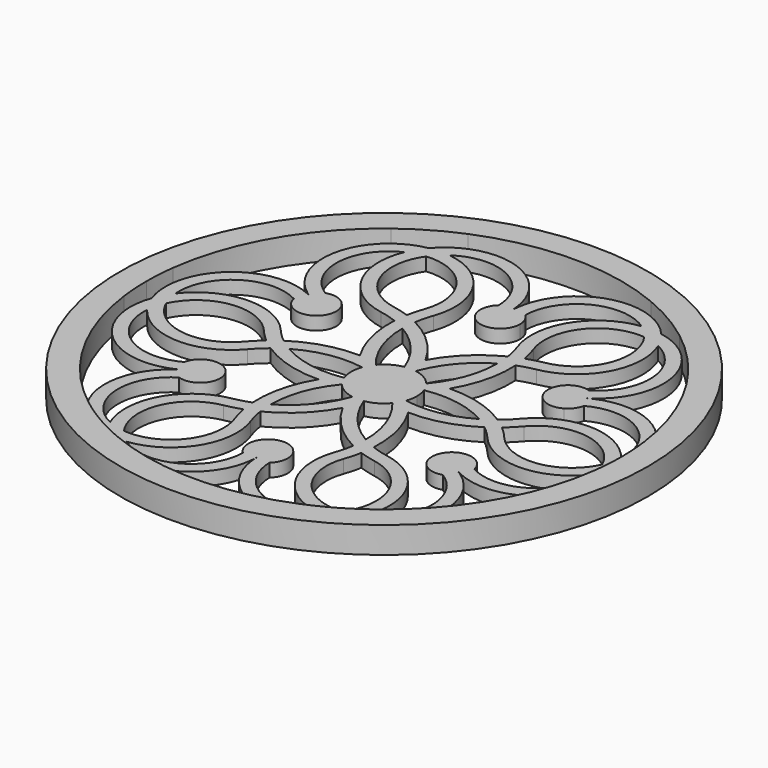
from build123d import *

# Parameters (mm, degrees)
F0_R     = 20
F2_DEPTH = 2
F3_DEPTH = 1
F4_COUNT = 6
F5_DEPTH = 1


# Not quite as in the source:
# - a feature names something its author has since deleted; it is built from what else it names


with BuildPart() as f2:
    # F0 (on Top) → F2 (new body)
    with BuildSketch(Plane.XY):
        Circle(F0_R)
        with BuildLine():
            ThreePointArc((18, 0), (-9.9846036052, -14.9769052493), (-6.9230767608, 16.615384683))
            ThreePointArc((-6.9230767608, 16.615384683), (1.3e-07, 18), (6.9230770009, 16.615384583))
            ThreePointArc((6.9230770009, 16.615384583), (14.9769053214, 9.984603497), (18, 0))
        make_face(mode=Mode.SUBTRACT)
    extrude(amount=F2_DEPTH)

    # F0 (on Top) → F3 (join)
    with BuildSketch(Plane.XY):
        with BuildLine():
            ThreePointArc((-1.0016972865, 12.1165135674), (-0.5479723364, 12.3963260072), (-0.0250418091, 12.4997909547))
            ThreePointArc((-0.0250418091, 12.4997909547), (-2.4381602314, 16.2938301084), (-6.9230767608, 16.615384683))
            ThreePointArc((-6.9230767608, 16.615384683), (-9.971545779, 11.4673344692), (-5.9016393443, 7.0819672131))
            ThreePointArc((-5.9016393443, 7.0819672131), (-2.5530323929, 5.499608355), (-0.4340277778, 2.4620357203))
            ThreePointArc((-0.4340277778, 2.4620357203), (0, 2.5), (0.4340277778, 2.4620357203))
            ThreePointArc((0.4340277778, 2.4620357203), (2.5530323929, 5.499608355), (5.9016393443, 7.0819672131))
            ThreePointArc((5.9016393443, 7.0819672131), (9.9715457651, 11.4673343399), (6.9230770009, 16.615384583))
            ThreePointArc((6.9230770009, 16.615384583), (2.4381603431, 16.293830175), (0.0250418091, 12.4997909547))
            ThreePointArc((0.0250418091, 12.4997909547), (0.5479723364, 12.3963260072), (1.0016972865, 12.1165135674))
            ThreePointArc((1.0016972865, 12.1165135674), (7.6052247894, 15.0352600872), (5.7213114754, 8.0655737705))
            ThreePointArc((5.7213114754, 8.0655737705), (2.3919359235, 6.6424784408), (0, 3.9242833741))
            ThreePointArc((0, 3.9242833741), (-2.3919359235, 6.6424784408), (-5.7213114754, 8.0655737705))
            ThreePointArc((-5.7213114754, 8.0655737705), (-7.6052247894, 15.0352600872), (-1.0016972865, 12.1165135674))
        make_face()
        with BuildLine():
            ThreePointArc((0.0250418091, 12.4997909547), (0.0062643765, 12.250208958), (0, 12))
            ThreePointArc((0, 12), (-0.0062643765, 12.250208958), (-0.0250418091, 12.4997909547))
            ThreePointArc((-0.0250418091, 12.4997909547), (-0.5479723364, 12.3963260072), (-1.0016972865, 12.1165135674))
            ThreePointArc((-1.0016972865, 12.1165135674), (-0.6113321807, 9.630228864), (1.5, 11))
            ThreePointArc((1.5, 11), (1.369771136, 11.6113321807), (1.0016972865, 12.1165135674))
            ThreePointArc((1.0016972865, 12.1165135674), (0.5479723364, 12.3963260072), (0.0250418091, 12.4997909547))
        make_face()
    extrude(amount=F3_DEPTH)

    # F4: F2 ×6 about axis
    f4_axis = Axis((0, 0, 6.8624988198), (0, 0, 1))


with BuildPart() as f2_1:
    add(f2.part)
    for i in range(1, F4_COUNT):
        add(f2.part.rotate(f4_axis, i * 360 / F4_COUNT))

    # F0 (on Top) → F5 (join)
    with BuildSketch(Plane.XY):
        with BuildLine():
            ThreePointArc((0, 0), (-0.1093371255, 1.25), (-0.4340277778, 2.4620357203))
            ThreePointArc((-0.4340277778, 2.4620357203), (-1.6070050646, -1.9150808657), (2.5, 0))
            ThreePointArc((2.5, 0), (1.9150808657, 1.6070050646), (0.4340277778, 2.4620357203))
            ThreePointArc((0.4340277778, 2.4620357203), (0.1093371255, 1.25), (0, 0))
        make_face()
        with BuildLine():
            ThreePointArc((0.4340277778, 2.4620357203), (0, 2.5), (-0.4340277778, 2.4620357203))
            ThreePointArc((-0.4340277778, 2.4620357203), (-0.1093371255, 1.25), (0, 0))
            ThreePointArc((0, 0), (0.1093371255, 1.25), (0.4340277778, 2.4620357203))
        make_face()
    extrude(amount=F5_DEPTH)


solid = f2_1.part
